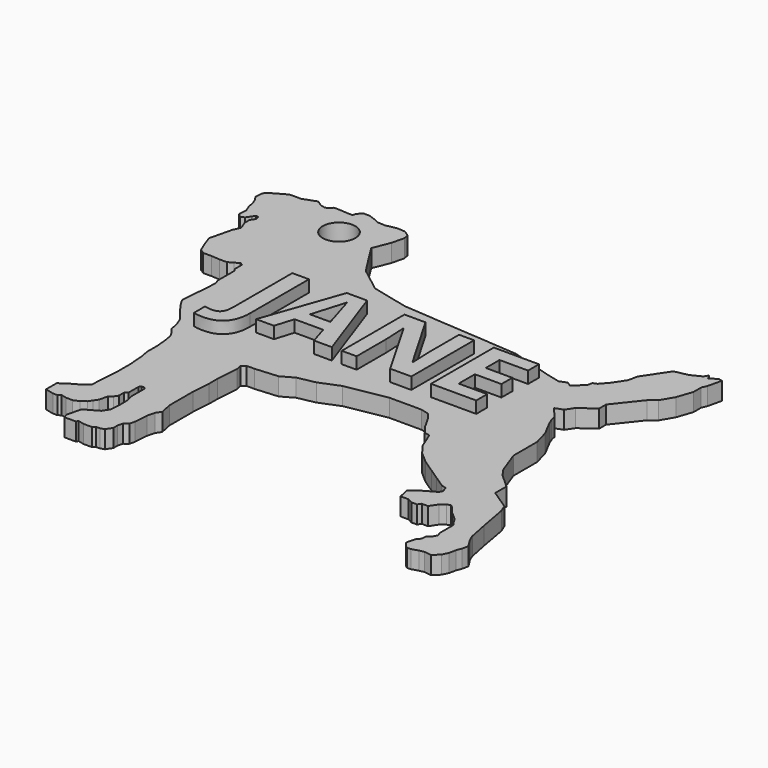
from build123d import *

# Parameters (mm, degrees)
F1_DEPTH     = 3
F2_TEXT_SIZE = 18.5588788655
F3_DEPTH     = 2
F4_R         = 2.75
F5_DEPTH     = 25


# Not quite as in the source:
# - Text() gives the source's letters only with a copy of the font that has no kerning and outlines rounded to 1/6400 em; it was checked with that copy


with BuildPart() as f1:
    # F0 (on Top) → F1 (new body)
    with BuildSketch(Plane.XY):
        Polygon((-4.4858887895, 1.2453554889), (-3.6428940416, 1.4245910626), (-2.4296078457, 1.2453554889), (-1.4231319801, 2.2242566838), (-0.9405755433, 3.2169451713), (-0.7061905424, 4.4026564392), (-0.3615072447, 5.257471659), (-0.1546971717, 6.3053093163), (-1.1335978951, 7.8494915603), (-1.5354520983, 8.8431066997), (-2.2200001548, 12.2099729866), (-3.0649793853, 16.8837643069), (-3.5881149826, 18.1772569354), (-6.8834482622, 20.375553711), (-6.8834482622, 22.7363859381), (-9.3081927281, 24.951195367), (-10.2448218553, 26.2950561598), (-11.6798182906, 30.2199013955), (-11.6798182906, 35.2455625824), (-12.4019250759, 37.8183820619), (-13.7718487283, 40.4289096251), (-14.2280614718, 41.5569303979), (-14.353108804, 42.2485984469), (-15.9899203014, 44.1521000185), (-14.6509958204, 44.6416357179), (-13.7773102535, 45.9513247265), (-11.251187891, 47.7722790825), (-11.251187891, 49.2383070429), (-7.791689326, 53.6056131825), (-6.6111771863, 54.5237929493), (-5.3762281847, 56.6356486643), (-4.4858887895, 59.2381758804), (-4.4858887895, 60.8818795904), (-4.1092064606, 61.7379771017), (-3.5619052729, 64.0915442673), (-4.136849206, 64.225242384), (-5.4110722896, 63.5094010325), (-5.8002980322, 64.2022367074), (-6.2639478797, 63.5072073603), (-7.9793593365, 62.6533035211), (-10.2448218553, 62.1926918329), (-12.2599435034, 59.1719452699), (-13.0057477291, 58.0539554188), (-13.3213970799, 56.4894146086), (-14.6548590763, 54.4905026589), (-15.8160046602, 53.1556018824), (-16.470396766, 52.8909418467), (-16.6721007997, 52.0597957509), (-18.3326488622, 50.4798094839), (-19.0979651008, 50.990347289), (-20.2767178563, 50.5136166812), (-22.7510637039, 51.1140953948), (-29.5857284677, 53.1258941459), (-35.9385172108, 53.6056131825), (-42.7351578647, 54.0848219089), (-49.5462635823, 54.5991499001), (-55.7600004357, 56.1071107682), (-59.8388219759, 59.2381758804), (-62.2259049994, 62.972395559), (-63.3485545455, 64.7860325701), (-62.208313015, 67.6366418835), (-61.7054206363, 69.7088713249), (-61.8680801525, 70.6085817647), (-62.8556613768, 71.2673911891), (-64.0836264356, 71.3539709572), (-65.2234646478, 71.1478985099), (-66.0497542461, 70.9798980934), (-67.3197635507, 71.0694422627), (-68.390062785, 71.5632265637), (-69.2862388534, 71.8702785029), (-70.2651400483, 71.8702785029), (-70.7063334074, 71.5080801374), (-71.0586804345, 70.9798980934), (-71.1487921509, 70.6085817647), (-72.043708322, 70.6085817647), (-73.5755472572, 70.7242557353), (-74.4047326014, 70.7242557353), (-74.7138275791, 70.2609102134), (-75.392793186, 69.9863117576), (-76.1342131623, 70.1662408948), (-77.1190390817, 70.8232122721), (-78.4419472565, 70.3395324322), (-79.3572303054, 70.0048879217), (-81.3219875434, 70.0048879217), (-83.9834254094, 68.4964377721), (-84.3237730532, 67.9862432752), (-84.4475772409, 66.7103465381), (-83.9196366327, 65.9448757309), (-83.6109023326, 65.1004594542), (-83.3866720911, 63.9976103069), (-82.9722214749, 62.9728495763), (-83.0715986629, 61.5633780898), (-82.4950151333, 60.9693401763), (-81.8141726164, 61.244697723), (-81.332751976, 61.9663661871), (-80.9661719225, 62.5158840972), (-80.5054078417, 62.404065039), (-80.3835217986, 61.8045833731), (-80.9020799559, 61.0272443113), (-80.9020799559, 59.973697514), (-80.3588205618, 58.6304472648), (-80.9020799559, 57.4488691434), (-81.3153612625, 55.745893065), (-81.834768245, 53.6056131825), (-81.2695886339, 52.0597957509), (-80.5944102527, 50.3903657535), (-79.8041505752, 49.8631883321), (-78.3725536392, 49.8631883321), (-76.9293358759, 49.7614318054), (-75.7359398958, 49.7614318054), (-74.8935632338, 50.2388741752), (-74.1135369684, 50.6809775779), (-73.67789842, 50.3903657535), (-73.67789842, 48.9062048382), (-73.3803548565, 48.3812330935), (-73.3803548565, 44.8875009336), (-73.0886076753, 44.1661337964), (-73.2954244975, 41.2328407564), (-73.5672831883, 37.6326900454), (-73.0521797344, 36.7238659538), (-72.103469489, 35.3704843277), (-71.2529469796, 34.2435465296), (-70.3528036609, 33.1434905566), (-69.8316491655, 31.854896354), (-69.5338441022, 30.3901784013), (-68.7368213186, 29.3161529821), (-68.3959746716, 28.7147793317), (-68.1488554186, 27.4993533676), (-67.9477664974, 25.362242013), (-67.9477664974, 23.1508922679), (-67.6877002309, 21.8717879937), (-67.4665988383, 19.0593868499), (-67.4665988383, 16.3924206232), (-67.5880604355, 14.6697248874), (-67.7386302486, 12.5341859105), (-67.7386302486, 11.3265375261), (-68.9319660245, 10.425903134), (-70.7262874488, 9.4089173702), (-71.6449307167, 8.7155989113), (-71.6449307167, 6.4966996528), (-70.1880818091, 6.143148932), (-69.4526383934, 6.143148932), (-68.9969643275, 6.4870552689), (-68.0480589343, 6.2567731964), (-67.5880604355, 6.2567731964), (-66.9705114644, 6.2567731964), (-66.0497542461, 6.6291609989), (-65.234230184, 7.2446533295), (-64.8307462813, 7.8494915603), (-64.3501863698, 8.5698697579), (-63.9927036661, 10.042920881), (-63.4197114527, 10.4753695717), (-63.0253639356, 11.0665120013), (-63.0253639356, 12.2267158257), (-62.5646329604, 12.5744387133), (-62.5646329604, 14.6697248874), (-62.3299590414, 15.0215103168), (-61.8680801525, 15.0215103168), (-61.6025806487, 14.6697248874), (-61.6025806487, 12.0946881479), (-61.2820132952, 10.5180166418), (-61.2820132952, 9.2692877474), (-61.3295587574, 8.5949481467), (-61.4221868898, 7.2811988426), (-62.1145325888, 6.2433454245), (-64.4278659298, 4.9321940093), (-65.0289474923, 2.4553640491), (-64.7554891006, 1.7792173377), (-63.8091506671, 1.7792173377), (-62.8585469966, 1.7792173377), (-62.634927237, 2.1144321477), (-61.6121316218, 1.8662182628), (-60.2179879516, 1.8662182628), (-59.7666923694, 2.2068200705), (-59.1617665285, 2.2370684539), (-58.4752182138, 2.4553640491), (-57.8241505579, 3.4313400581), (-57.8241505579, 4.3231114917), (-57.6167724019, 5.1776385011), (-56.9297172488, 5.6961727751), (-56.7032979837, 6.6291609989), (-56.5417084224, 8.9209935985), (-56.2317495685, 10.1982168969), (-55.6603464243, 11.0547726714), (-56.0802331736, 13.1199345357), (-56.0802331736, 15.0437873324), (-56.0802331736, 18.107817431), (-55.8637986754, 21.177518437), (-55.8637986754, 22.9132523247), (-55.5951372555, 26.7236902994), (-55.8076509087, 27.7689128339), (-55.1693332906, 28.2506639148), (-53.8447511331, 28.2506639148), (-50.0159429872, 28.5525862355), (-47.9726666791, 29.7106746854), (-45.0530647841, 30.3042853704), (-41.7270278822, 31.6494560064), (-34.7995198006, 32.9018868589), (-31.1558542245, 32.9018868589), (-29.3850860149, 32.9018868589), (-27.9545231514, 32.5547152827), (-27.0636371909, 31.3742961269), (-25.9448293729, 29.4003247017), (-24.9068945179, 28.0250665433), (-23.9561996392, 27.7943501953), (-22.8063241263, 24.951195367), (-21.5348886561, 23.2665501362), (-19.6538159403, 21.6198669736), (-17.4899703535, 20.1763787516), (-15.6666388556, 18.960045406), (-13.6767852491, 17.6326261752), (-12.9106253628, 17.446693112), (-12.5686731762, 16.5114229068), (-12.8330795905, 15.9796413917), (-14.0227813012, 15.3053420791), (-15.1442341134, 14.6697248874), (-16.421459266, 13.7057775038), (-16.0402045023, 11.8306223583), (-15.1704718429, 11.8306223583), (-14.6548590763, 11.8306223583), (-13.8501923204, 11.3867596185), (-12.8995900217, 11.3867596185), (-12.5337901773, 11.9351079644), (-11.4736879454, 11.9148710159), (-10.6201854854, 13.1943047538), (-9.8133827277, 13.8032149414), (-9.3081927281, 14.0273193493), (-8.8087682272, 13.6941563042), (-7.9636949525, 12.5744387133), (-6.4038115337, 11.2283254448), (-5.9741090372, 10.4701787499), (-5.4639964563, 9.7942822954), (-5.4639964563, 8.2180871184), (-5.4639964563, 6.8403407671), (-5.2233920368, 6.2454280054), (-5.5504439076, 5.5733187001), (-6.2353206821, 4.9321940093), (-6.2896891925, 4.1610827839), (-6.8174659747, 3.5186887196), (-7.0229289384, 2.799568518), (-7.1941476176, 2.2516669955), (-7.1599047048, 1.8749848382), (-6.6847108342, 1.2453554889), (-6.1698120636, 0.9018696526), (-5.5655176071, 0.9264955426), align=None)
    extrude(amount=F1_DEPTH)

    # F2 (on face) → F3 (join)
    with BuildSketch(Plane.XY.offset(3)):
        with Locations((-66.2808343768, 36.4454239607)):
            Text('JANE', F2_TEXT_SIZE, font='Open Sans', font_style=FontStyle.BOLD, text_align=(TextAlign.LEFT, TextAlign.BOTTOM))
    extrude(amount=F3_DEPTH)

    # F4 (on face) → F5 (cut)
    with BuildSketch(Plane.XY.offset(3)):
        with Locations((-69.522626698, 65.6942054629)):
            Circle(F4_R)
    extrude(amount=-F5_DEPTH, mode=Mode.SUBTRACT)


solid = f1.part
